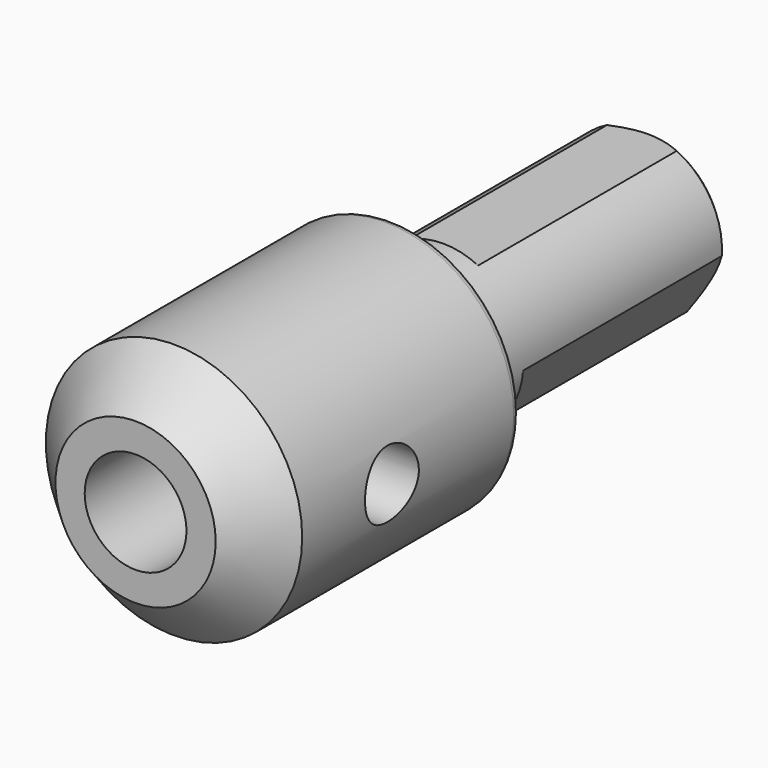
from build123d import *

# Parameters (mm, degrees)
F0_R            = 8
F1_DEPTH        = 20
F2_R            = 5
F3_DEPTH        = 20
F5_DEPTH        = 16
F5_COPIES_COUNT = 3
F6_SIZE         = 0.49999
F7_R            = 0.5
F9_D            = 6.35
F9_DEPTH        = 14
F9_TIP          = 1.9077324654
F10_R           = 2.1
F11_DEPTH       = 8.25
F12_SIZE        = 3


# Not quite as in the source:
# - a fillet or chamfer is up to 0.001 mm smaller than in the source, because OpenCascade refuses the exact size
# - a pattern or mirror of a feature is missing from the dataset's text; its kind, count and spacing are read off the source's solid


with BuildPart() as f1:
    # F0 (on Front) → F1 (new body)
    with BuildSketch(Plane.XZ):
        Circle(F0_R)
    extrude(amount=-F1_DEPTH)

    # F2 (on face) → F3 (join)
    with BuildSketch(Plane(origin=(0, 20, 0), x_dir=(-1, 0, 0), z_dir=(0, 1, 0))):
        Circle(F2_R)
    extrude(amount=F3_DEPTH)

    # F4 (on face) → F5 (cut)
    with BuildSketch(Plane(origin=(0, 40, 0), x_dir=(-1, 0, 0), z_dir=(0, 1, 0))):
        with BuildLine():
            ThreePointArc((2.1794494718, 4.5), (0, 5), (-2.1794494718, 4.5))
            Line((-2.1794494718, 4.5), (2.1794494718, 4.5))
        make_face()
    f5 = extrude(amount=-F5_DEPTH, mode=Mode.SUBTRACT)

    # F5_copies: F5 ×3 about axis
    f5_copies_axis = Axis((0, 0, 0), (0, 1, 0))
    for i in range(1, F5_COPIES_COUNT):
        add(f5.rotate(f5_copies_axis, i * 360 / F5_COPIES_COUNT), mode=Mode.SUBTRACT)

    # F6 (size 0.5 in the source; OpenCascade refuses exactly that, so slightly less here)
    f6_edges = [f1.edges().sort_by_distance(p)[0] for p in [
        (4.330127, 40, 2.5),
        (-4.996709, 40, -0.18139),
        (0, 40, -5),
        (-4.236582, 40, 2.655443),
    ]]
    chamfer(f6_edges, length=F6_SIZE)

    # F7
    f7_edges = [f1.edges().sort_by_distance(p)[0] for p in [
        (-8, 20, 0),
        (5, 20, 0),
    ]]
    fillet(f7_edges, radius=F7_R)

    # F9
    with Locations(Plane.XZ):
        with Locations((0, 0)):
            Hole(F9_D / 2, depth=F9_DEPTH)
            with Locations((0, 0, -(F9_DEPTH + F9_TIP / 2))):  # 118° drill point
                Cone(0, F9_D / 2, F9_TIP, mode=Mode.SUBTRACT)

    # F10 (on Right) → F11 (cut, symmetric)
    with BuildSketch(Plane.YZ):
        with Locations((10, 0)):
            Circle(F10_R)
    extrude(amount=F11_DEPTH, both=True, mode=Mode.SUBTRACT)

    # F12
    f12_edges = [f1.edges().sort_by_distance(p)[0] for p in [
        (-8, 0, 0),
    ]]
    chamfer(f12_edges, length=F12_SIZE)


solid = f1.part
